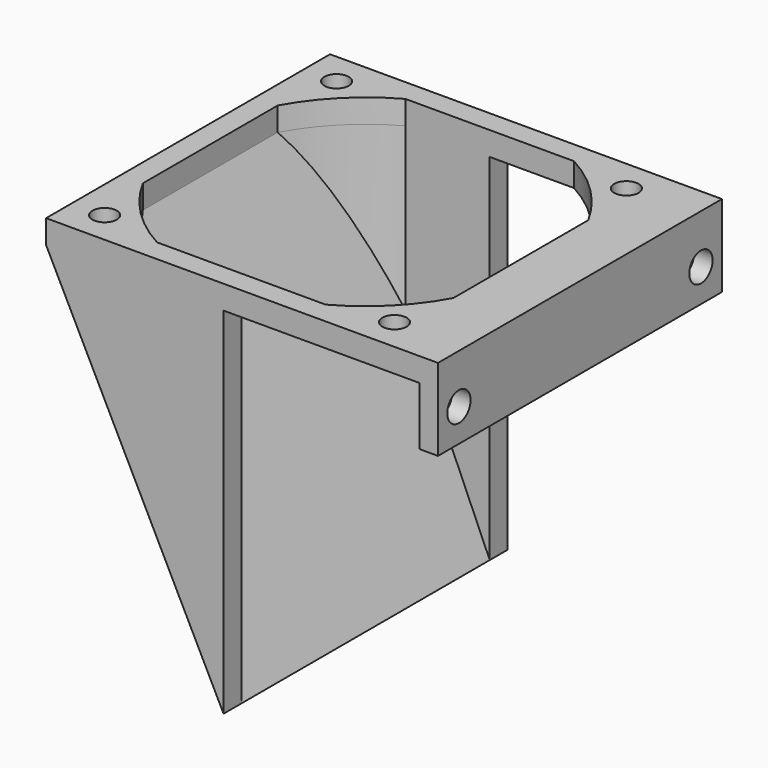
from build123d import *

# Parameters (mm, degrees)
F0_W        = 60.96
F0_H        = 4.064
F1_DEPTH    = 60.96
F3_DEPTH    = 25.4
F6_DEPTH    = 60.96
F7_T4_DEPTH = 53.34
F7_S5_R     = 30.988
F7_T6_DEPTH = 44
F7_S7_R     = 30.48
F7_T8_DEPTH = 44
F8_W        = 60.96
F8_H        = 4.064
F9_DEPTH    = 6.35
F10_W       = 3.175
F10_H       = 60.96
F11_DEPTH   = 10
F4_R        = 2.0955
F14_DEPTH   = 65.025
F13_R       = 2.5
F15_DEPTH   = 25.4
F12_R       = 2.5
F16_DEPTH   = 25.4


# Not quite as in the source:
# - a fillet or chamfer that OpenCascade refuses, or shapes differently, is made with other operations: its cross-section is extruded or revolved along the edge and cut away or added


with BuildPart() as f1:
    # F0 (on Right) → F1 (new body)
    with BuildSketch(Plane.YZ):
        with Locations((2.5902520865, 22.5415869818)):
            Rectangle(F0_W, F0_H)
    extrude(amount=F1_DEPTH)

    # F2 (on face) → F3 (cut)
    with BuildSketch(Plane.XY.offset(24.5735869818)):
        with BuildLine():
            Line((16.002, -24.0797479135), (44.958, -24.0797479135))
            ThreePointArc((44.958, -24.0797479135), (51.934072902, -18.8638208155), (57.15, -11.8877479135))
            Line((57.15, -11.8877479135), (57.15, 17.0682520865))
            ThreePointArc((57.15, 17.0682520865), (51.934072902, 24.0443249885), (44.958, 29.2602520865))
            Line((44.958, 29.2602520865), (16.002, 29.2602520865))
            ThreePointArc((16.002, 29.2602520865), (9.0409528702, 24.0292992163), (3.81, 17.0682520865))
            Line((3.81, 17.0682520865), (3.81, -11.8877479135))
            ThreePointArc((3.81, -11.8877479135), (9.025927098, -18.8638208155), (16.002, -24.0797479135))
        make_face()
    extrude(amount=-F3_DEPTH, mode=Mode.SUBTRACT)

    # F5 (on face) → F6 (join)
    with BuildSketch(Plane.XZ.offset(27.8897479135)):
        Polygon((30.48, -40.4504130182), (30.48, 20.5095869818), (0, 20.5095869818), align=None)
    extrude(amount=-F6_DEPTH)

    # F7: chamfer of 60.96 x 26.67 on 1 edges, made by hand


with BuildPart() as f7_tool2:
    # F7_s3 → F7_t4 (new body)
    with BuildSketch(Plane.XZ.offset(24.0797479135)):
        Polygon((3.81, 20.5095869818), (30.48, -40.4504130182), (30.48, 20.5095869818), align=None)
    extrude(amount=-F7_T4_DEPTH)

    # F7_s5 → F7_t6 (intersect, symmetric)
    with BuildSketch(Plane.XY.offset(-10)):
        with Locations((30.9527778056, 2.1174742809)):
            Circle(F7_S5_R)
    extrude(amount=F7_T6_DEPTH, both=True, mode=Mode.INTERSECT)

    # F7_s7 → F7_t8 (intersect, symmetric)
    with BuildSketch(Plane.XY.offset(-10)):
        with Locations((30.5785417886, 2.6887938751)):
            Circle(F7_S7_R)
    extrude(amount=F7_T8_DEPTH, both=True, mode=Mode.INTERSECT)


with BuildPart() as f1_1:
    add(f1.part)

    # F7_t1: cut F7_tool2
    add(f7_tool2.part, mode=Mode.SUBTRACT)

    # F8 (on face) → F9 (join)
    with BuildSketch(Plane.YZ.offset(60.96)):
        with Locations((2.5902520865, 22.5415869818)):
            Rectangle(F8_W, F8_H)
    extrude(amount=F9_DEPTH)

    # F10 (on face) → F11 (join)
    with BuildSketch(Plane(origin=(0, 0, 20.5095869818), x_dir=(1, 0, 0), z_dir=(0, 0, -1))):
        with Locations((65.7225, -2.5902520865)):
            Rectangle(F10_W, F10_H)
    extrude(amount=F11_DEPTH)

    # F4 (on face) → F14 (cut, through all)
    with BuildSketch(Plane.XY.offset(24.5735869818)):
        with Locations((55.372, -22.3017479135)):
            Circle(F4_R)
        with Locations((55.372, 27.4822520865)):
            Circle(F4_R)
        with Locations((5.588, -22.3017479135)):
            Circle(F4_R)
        with Locations((5.588, 27.4822520865)):
            Circle(F4_R)
    extrude(amount=-F14_DEPTH, mode=Mode.SUBTRACT)

    # F13 (on face) → F15 (cut)
    with BuildSketch(Plane(origin=(64.135, 0, 0), x_dir=(0, -1, 0), z_dir=(-1, 0, 0))):
        with Locations((23.3897479135, 16.1365869818)):
            Circle(F13_R)
    extrude(amount=-F15_DEPTH, mode=Mode.SUBTRACT)

    # F12 (on face) → F16 (cut)
    with BuildSketch(Plane(origin=(64.135, 0, 0), x_dir=(0, -1, 0), z_dir=(-1, 0, 0))):
        with Locations((-28.5702520865, 16.1365869818)):
            Circle(F12_R)
    extrude(amount=-F16_DEPTH, mode=Mode.SUBTRACT)


solid = f1_1.part
